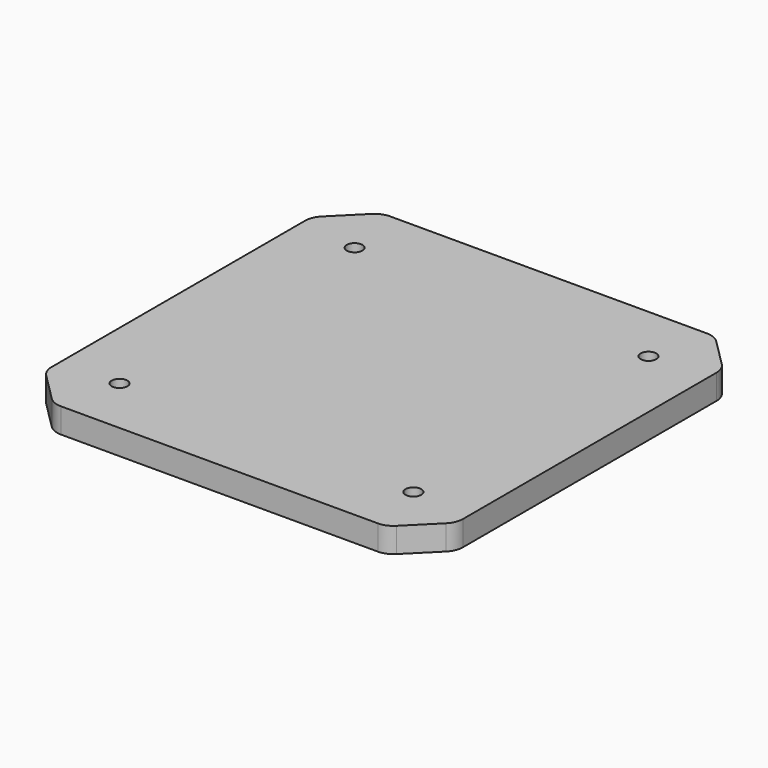
from build123d import *

# Parameters (mm, degrees)
F0_W     = 105
F0_H     = 105
F0_R     = 2
F1_DEPTH = 6.35
F2_SIZE  = 10
F3_R     = 5


# Not quite as in the source:
# - a length typed as a fraction of an inch, garbled in the dataset ("3 / 203.2 mm" for 3/8 in), is restored


with BuildPart() as f1:
    # F0 (on Top) → F1 (new body)
    with BuildSketch(Plane.XY):
        Rectangle(F0_W, F0_H)
        with Locations((-37.5, -37.5)):
            Circle(F0_R, mode=Mode.SUBTRACT)
        with Locations((37.5, -37.5)):
            Circle(F0_R, mode=Mode.SUBTRACT)
        with Locations((-37.5, 37.5)):
            Circle(F0_R, mode=Mode.SUBTRACT)
        with Locations((37.5, 37.5)):
            Circle(F0_R, mode=Mode.SUBTRACT)
    extrude(amount=F1_DEPTH)

    # F2
    f2_edges = [f1.edges().sort_by_distance(p)[0] for p in [
        (-52.5, -52.5, 3.175),
        (52.5, -52.5, 3.175),
        (52.5, 52.5, 3.175),
        (-52.5, 52.5, 3.175),
    ]]
    chamfer(f2_edges, length=F2_SIZE)

    # F3
    f3_edges = [f1.edges().sort_by_distance(p)[0] for p in [
        (52.5, 42.5, 3.175),
        (42.5, 52.5, 3.175),
        (-42.5, 52.5, 3.175),
        (-52.5, 42.5, 3.175),
        (-52.5, -42.5, 3.175),
        (-42.5, -52.5, 3.175),
        (42.5, -52.5, 3.175),
        (52.5, -42.5, 3.175),
    ]]
    fillet(f3_edges, radius=F3_R)


solid = f1.part
